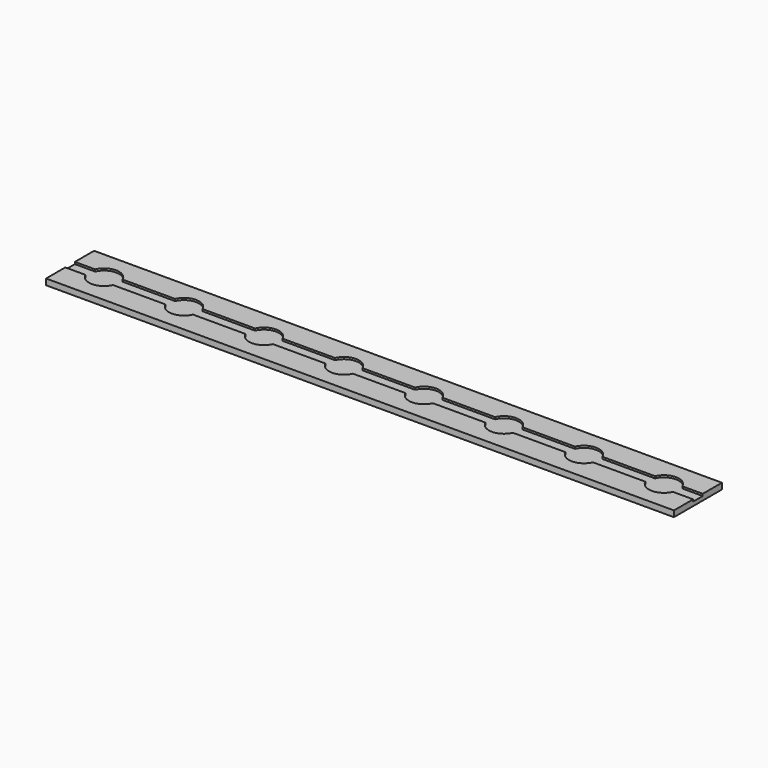
from build123d import *

# Parameters (mm, degrees)
F0_W     = 398.78
F0_H     = 38.1
F1_DEPTH = 3.81
F2_R     = 9.525
F3_DEPTH = 1.27
F5_DEPTH = 1.27


with BuildPart() as f1:
    # F0 (on Top) → F1 (new body)
    with BuildSketch(Plane.XY):
        with Locations((85.0978558012, 21.4591654949)):
            Rectangle(F0_W, F0_H)
    extrude(amount=F1_DEPTH)

    # F2 (on face) → F3 (cut)
    with BuildSketch(Plane.XY.offset(3.81)):
        with Locations((-92.7021441988, 21.4591654949)):
            Circle(F2_R)
        with Locations((-41.9021441988, 21.4591654949)):
            Circle(F2_R)
        with Locations((8.8978558012, 21.4591654949)):
            Circle(F2_R)
        with Locations((59.6978558012, 21.4591654949)):
            Circle(F2_R)
        with Locations((110.4978558012, 21.4591654949)):
            Circle(F2_R)
        with Locations((161.2978558012, 21.4591654949)):
            Circle(F2_R)
        with Locations((212.0978558012, 21.4591654949)):
            Circle(F2_R)
        with Locations((262.8978558012, 21.4591654949)):
            Circle(F2_R)
    extrude(amount=-F3_DEPTH, mode=Mode.SUBTRACT)

    # F4 (on face) → F5 (cut)
    with BuildSketch(Plane.XY.offset(3.81)):
        with BuildLine():
            Line((-101.4319508977, 25.2691654949), (-114.2921441988, 25.2691654949))
            Line((-114.2921441988, 25.2691654949), (-114.2921441988, 17.6491654949))
            Line((-114.2921441988, 17.6491654949), (-101.4319508977, 17.6491654949))
            ThreePointArc((-101.4319508977, 17.6491654949), (-102.2271441988, 21.4591654949), (-101.4319508977, 25.2691654949))
        make_face()
        with BuildLine():
            Line((-83.9723374999, 25.2691654949), (-101.4319508977, 25.2691654949))
            ThreePointArc((-101.4319508977, 25.2691654949), (-102.2271441988, 21.4591654949), (-101.4319508977, 17.6491654949))
            Line((-101.4319508977, 17.6491654949), (-83.9723374999, 17.6491654949))
            ThreePointArc((-83.9723374999, 17.6491654949), (-83.3780615681, 19.5131161387), (-83.1771441988, 21.4591654949))
            ThreePointArc((-83.1771441988, 21.4591654949), (-83.3780615681, 23.405214851), (-83.9723374999, 25.2691654949))
        make_face()
        with BuildLine():
            Line((-50.6319508977, 25.2691654949), (-83.9723374999, 25.2691654949))
            ThreePointArc((-83.9723374999, 25.2691654949), (-83.3780615681, 23.405214851), (-83.1771441988, 21.4591654949))
            ThreePointArc((-83.1771441988, 21.4591654949), (-83.3780615681, 19.5131161387), (-83.9723374999, 17.6491654949))
            Line((-83.9723374999, 17.6491654949), (-50.6319508977, 17.6491654949))
            ThreePointArc((-50.6319508977, 17.6491654949), (-51.4271441988, 21.4591654949), (-50.6319508977, 25.2691654949))
        make_face()
        with BuildLine():
            Line((-33.1723374999, 25.2691654949), (-50.6319508977, 25.2691654949))
            ThreePointArc((-50.6319508977, 25.2691654949), (-51.4271441988, 21.4591654949), (-50.6319508977, 17.6491654949))
            Line((-50.6319508977, 17.6491654949), (-33.1723374999, 17.6491654949))
            ThreePointArc((-33.1723374999, 17.6491654949), (-32.5780615681, 19.5131161387), (-32.3771441988, 21.4591654949))
            ThreePointArc((-32.3771441988, 21.4591654949), (-32.5780615681, 23.405214851), (-33.1723374999, 25.2691654949))
        make_face()
        with BuildLine():
            Line((284.4878558012, 17.6491654949), (284.4878558012, 25.2691654949))
            Line((284.4878558012, 25.2691654949), (271.6276625001, 25.2691654949))
            ThreePointArc((271.6276625001, 25.2691654949), (272.2219384319, 23.405214851), (272.4228558012, 21.4591654949))
            ThreePointArc((272.4228558012, 21.4591654949), (272.2219384319, 19.5131161387), (271.6276625001, 17.6491654949))
            Line((271.6276625001, 17.6491654949), (284.4878558012, 17.6491654949))
        make_face()
        with BuildLine():
            Line((0.1680491023, 25.2691654949), (-33.1723374999, 25.2691654949))
            ThreePointArc((-33.1723374999, 25.2691654949), (-32.5780615681, 23.405214851), (-32.3771441988, 21.4591654949))
            ThreePointArc((-32.3771441988, 21.4591654949), (-32.5780615681, 19.5131161387), (-33.1723374999, 17.6491654949))
            Line((-33.1723374999, 17.6491654949), (0.1680491023, 17.6491654949))
            ThreePointArc((0.1680491023, 17.6491654949), (-0.6271441988, 21.4591654949), (0.1680491023, 25.2691654949))
        make_face()
        with BuildLine():
            Line((17.6276625001, 25.2691654949), (0.1680491023, 25.2691654949))
            ThreePointArc((0.1680491023, 25.2691654949), (-0.6271441988, 21.4591654949), (0.1680491023, 17.6491654949))
            Line((0.1680491023, 17.6491654949), (17.6276625001, 17.6491654949))
            ThreePointArc((17.6276625001, 17.6491654949), (18.2219384319, 19.5131161387), (18.4228558012, 21.4591654949))
            ThreePointArc((18.4228558012, 21.4591654949), (18.2219384319, 23.405214851), (17.6276625001, 25.2691654949))
        make_face()
        with BuildLine():
            ThreePointArc((254.1680491023, 17.6491654949), (253.3728558012, 21.4591654949), (254.1680491023, 25.2691654949))
            Line((254.1680491023, 25.2691654949), (220.8276625001, 25.2691654949))
            ThreePointArc((220.8276625001, 25.2691654949), (221.4219384319, 23.405214851), (221.6228558012, 21.4591654949))
            ThreePointArc((221.6228558012, 21.4591654949), (221.4219384319, 19.5131161387), (220.8276625001, 17.6491654949))
            Line((220.8276625001, 17.6491654949), (254.1680491023, 17.6491654949))
        make_face()
        with BuildLine():
            Line((50.9680491023, 25.2691654949), (17.6276625001, 25.2691654949))
            ThreePointArc((17.6276625001, 25.2691654949), (18.2219384319, 23.405214851), (18.4228558012, 21.4591654949))
            ThreePointArc((18.4228558012, 21.4591654949), (18.2219384319, 19.5131161387), (17.6276625001, 17.6491654949))
            Line((17.6276625001, 17.6491654949), (50.9680491023, 17.6491654949))
            ThreePointArc((50.9680491023, 17.6491654949), (50.1728558012, 21.4591654949), (50.9680491023, 25.2691654949))
        make_face()
        with BuildLine():
            ThreePointArc((221.6228558012, 21.4591654949), (221.4219384319, 23.405214851), (220.8276625001, 25.2691654949))
            Line((220.8276625001, 25.2691654949), (203.3680491023, 25.2691654949))
            ThreePointArc((203.3680491023, 25.2691654949), (202.5728558012, 21.4591654949), (203.3680491023, 17.6491654949))
            Line((203.3680491023, 17.6491654949), (220.8276625001, 17.6491654949))
            ThreePointArc((220.8276625001, 17.6491654949), (221.4219384319, 19.5131161387), (221.6228558012, 21.4591654949))
        make_face()
        with BuildLine():
            Line((68.4276625001, 25.2691654949), (50.9680491023, 25.2691654949))
            ThreePointArc((50.9680491023, 25.2691654949), (50.1728558012, 21.4591654949), (50.9680491023, 17.6491654949))
            Line((50.9680491023, 17.6491654949), (68.4276625001, 17.6491654949))
            ThreePointArc((68.4276625001, 17.6491654949), (69.0219384319, 19.5131161387), (69.2228558012, 21.4591654949))
            ThreePointArc((69.2228558012, 21.4591654949), (69.0219384319, 23.405214851), (68.4276625001, 25.2691654949))
        make_face()
        with BuildLine():
            ThreePointArc((203.3680491023, 17.6491654949), (202.5728558012, 21.4591654949), (203.3680491023, 25.2691654949))
            Line((203.3680491023, 25.2691654949), (170.0276625001, 25.2691654949))
            ThreePointArc((170.0276625001, 25.2691654949), (170.6219384319, 23.405214851), (170.8228558012, 21.4591654949))
            ThreePointArc((170.8228558012, 21.4591654949), (170.6219384319, 19.5131161387), (170.0276625001, 17.6491654949))
            Line((170.0276625001, 17.6491654949), (203.3680491023, 17.6491654949))
        make_face()
        with BuildLine():
            Line((101.7680491023, 25.2691654949), (68.4276625001, 25.2691654949))
            ThreePointArc((68.4276625001, 25.2691654949), (69.0219384319, 23.405214851), (69.2228558012, 21.4591654949))
            ThreePointArc((69.2228558012, 21.4591654949), (69.0219384319, 19.5131161387), (68.4276625001, 17.6491654949))
            Line((68.4276625001, 17.6491654949), (101.7680491023, 17.6491654949))
            ThreePointArc((101.7680491023, 17.6491654949), (100.9728558012, 21.4591654949), (101.7680491023, 25.2691654949))
        make_face()
        with BuildLine():
            ThreePointArc((170.8228558012, 21.4591654949), (170.6219384319, 23.405214851), (170.0276625001, 25.2691654949))
            Line((170.0276625001, 25.2691654949), (152.5680491023, 25.2691654949))
            ThreePointArc((152.5680491023, 25.2691654949), (151.7728558012, 21.4591654949), (152.5680491023, 17.6491654949))
            Line((152.5680491023, 17.6491654949), (170.0276625001, 17.6491654949))
            ThreePointArc((170.0276625001, 17.6491654949), (170.6219384319, 19.5131161387), (170.8228558012, 21.4591654949))
        make_face()
        with BuildLine():
            Line((119.2276625001, 25.2691654949), (101.7680491023, 25.2691654949))
            ThreePointArc((101.7680491023, 25.2691654949), (100.9728558012, 21.4591654949), (101.7680491023, 17.6491654949))
            Line((101.7680491023, 17.6491654949), (119.2276625001, 17.6491654949))
            ThreePointArc((119.2276625001, 17.6491654949), (119.8219384319, 19.5131161387), (120.0228558012, 21.4591654949))
            ThreePointArc((120.0228558012, 21.4591654949), (119.8219384319, 23.405214851), (119.2276625001, 25.2691654949))
        make_face()
        with BuildLine():
            ThreePointArc((152.5680491023, 17.6491654949), (151.7728558012, 21.4591654949), (152.5680491023, 25.2691654949))
            Line((152.5680491023, 25.2691654949), (119.2276625001, 25.2691654949))
            ThreePointArc((119.2276625001, 25.2691654949), (119.8219384319, 23.405214851), (120.0228558012, 21.4591654949))
            ThreePointArc((120.0228558012, 21.4591654949), (119.8219384319, 19.5131161387), (119.2276625001, 17.6491654949))
            Line((119.2276625001, 17.6491654949), (152.5680491023, 17.6491654949))
        make_face()
    extrude(amount=-F5_DEPTH, mode=Mode.SUBTRACT)


solid = f1.part
